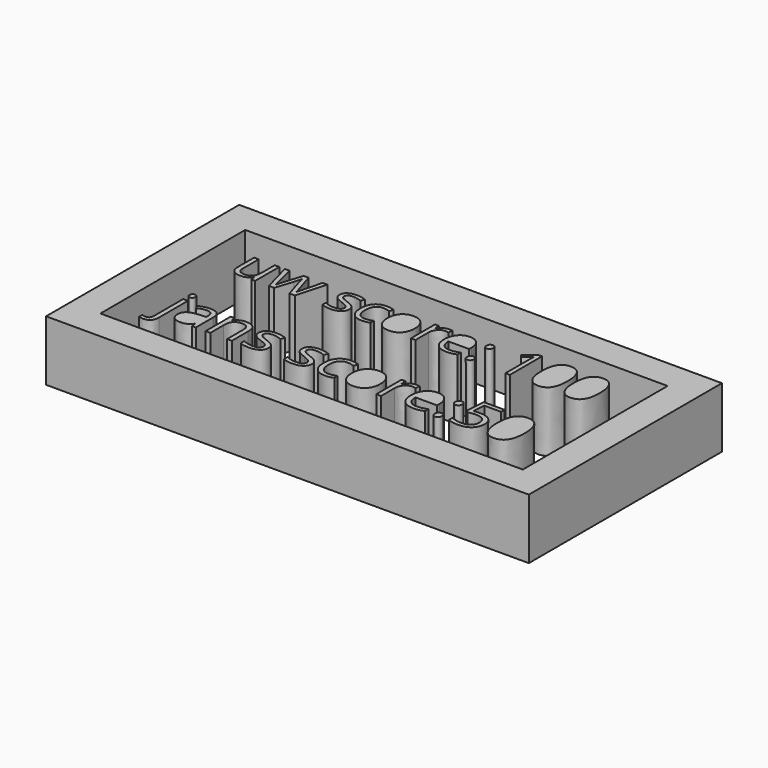
from build123d import *

# Parameters (mm, degrees)
F0_W           = 80
F0_H           = 40
F0_TEXT_SIZE   = 9.3251414556
F0_TEXT_SIZE_2 = 9.7321134399
F1_DEPTH       = 10


# Not quite as in the source:
# - Text() gives the source's letters only with a copy of the font that has no kerning and outlines rounded to 1/6400 em; it was checked with that copy


with BuildPart() as f1:
    # F0 (on Top) → F1 (new body)
    with BuildSketch(Plane.XY):
        with Locations((-35, -20.7777848959)):
            Rectangle(F0_W, F0_H)
        Polygon((-70, -20.7777848959), (-70, -5.7777848959), (0, -5.7777848959), (0, -20.7777848959), (0, -35.7777848959), (-70, -35.7777848959), align=None, mode=Mode.SUBTRACT)
        with BuildLine():
            add(Edge.make_bspline(
                [(-9.5991839217, -25.4409322699), (-9.9557746407, -26.1275024602), (-9.9557746407, -27.643583257)],
                knots=[0, 0, 0, 1, 1, 1], degree=2))
            add(Edge.make_bspline(
                [(-9.9557746407, -27.643583257), (-9.9557746407, -29.1596640539), (-9.5991839217, -29.8515564937)],
                knots=[0, 0, 0, 1, 1, 1], degree=2))
            add(Edge.make_bspline(
                [(-9.5991839217, -29.8515564937), (-9.2425932027, -30.5434489336), (-8.4640241275, -30.5434489336)],
                knots=[0, 0, 0, 1, 1, 1], degree=2))
            add(Edge.make_bspline(
                [(-8.4640241275, -30.5434489336), (-7.6748105533, -30.5434489336), (-7.3212611197, -29.8424326374)],
                knots=[0, 0, 0, 1, 1, 1], degree=2))
            add(Edge.make_bspline(
                [(-7.3212611197, -29.8424326374), (-6.9677116861, -29.1414163412), (-6.9677116861, -27.643583257)],
                knots=[0, 0, 0, 1, 1, 1], degree=2))
            add(Edge.make_bspline(
                [(-6.9677116861, -27.643583257), (-6.9677116861, -26.1472708156), (-7.3212611197, -25.4508164476)],
                knots=[0, 0, 0, 1, 1, 1], degree=2))
            add(Edge.make_bspline(
                [(-7.3212611197, -25.4508164476), (-7.6748105533, -24.7543620796), (-8.4640241275, -24.7543620796)],
                knots=[0, 0, 0, 1, 1, 1], degree=2))
            add(Edge.make_bspline(
                [(-8.4640241275, -24.7543620796), (-9.2425932027, -24.7543620796), (-9.5991839217, -25.4409322699)],
                knots=[0, 0, 0, 1, 1, 1], degree=2))
        make_face()
        with BuildLine():
            add(Edge.make_bspline(
                [(-14.2326185677, -10.6584024681), (-14.5742975789, -11.3162620568), (-14.5742975789, -12.7689442491)],
                knots=[0, 0, 0, 1, 1, 1], degree=2))
            add(Edge.make_bspline(
                [(-14.5742975789, -12.7689442491), (-14.5742975789, -14.2216264415), (-14.2326185677, -14.8845857169)],
                knots=[0, 0, 0, 1, 1, 1], degree=2))
            add(Edge.make_bspline(
                [(-14.2326185677, -14.8845857169), (-13.8909395566, -15.5475449922), (-13.1449282401, -15.5475449922)],
                knots=[0, 0, 0, 1, 1, 1], degree=2))
            add(Edge.make_bspline(
                [(-13.1449282401, -15.5475449922), (-12.3887175502, -15.5475449922), (-12.0499526458, -14.8758433968)],
                knots=[0, 0, 0, 1, 1, 1], degree=2))
            add(Edge.make_bspline(
                [(-12.0499526458, -14.8758433968), (-11.7111877413, -14.2041418013), (-11.7111877413, -12.7689442491)],
                knots=[0, 0, 0, 1, 1, 1], degree=2))
            add(Edge.make_bspline(
                [(-11.7111877413, -12.7689442491), (-11.7111877413, -11.3352037503), (-12.0499526458, -10.6678733149)],
                knots=[0, 0, 0, 1, 1, 1], degree=2))
            add(Edge.make_bspline(
                [(-12.0499526458, -10.6678733149), (-12.3887175502, -10.0005428795), (-13.1449282401, -10.0005428795)],
                knots=[0, 0, 0, 1, 1, 1], degree=2))
            add(Edge.make_bspline(
                [(-13.1449282401, -10.0005428795), (-13.8909395566, -10.0005428795), (-14.2326185677, -10.6584024681)],
                knots=[0, 0, 0, 1, 1, 1], degree=2))
        make_face()
        with BuildLine():
            add(Edge.make_bspline(
                [(-8.9012603511, -10.6584024681), (-9.2429393623, -11.3162620568), (-9.2429393623, -12.7689442491)],
                knots=[0, 0, 0, 1, 1, 1], degree=2))
            add(Edge.make_bspline(
                [(-9.2429393623, -12.7689442491), (-9.2429393623, -14.2216264415), (-8.9012603511, -14.8845857169)],
                knots=[0, 0, 0, 1, 1, 1], degree=2))
            add(Edge.make_bspline(
                [(-8.9012603511, -14.8845857169), (-8.55958134, -15.5475449922), (-7.8135700236, -15.5475449922)],
                knots=[0, 0, 0, 1, 1, 1], degree=2))
            add(Edge.make_bspline(
                [(-7.8135700236, -15.5475449922), (-7.0573593336, -15.5475449922), (-6.7185944292, -14.8758433968)],
                knots=[0, 0, 0, 1, 1, 1], degree=2))
            add(Edge.make_bspline(
                [(-6.7185944292, -14.8758433968), (-6.3798295248, -14.2041418013), (-6.3798295248, -12.7689442491)],
                knots=[0, 0, 0, 1, 1, 1], degree=2))
            add(Edge.make_bspline(
                [(-6.3798295248, -12.7689442491), (-6.3798295248, -11.3352037503), (-6.7185944292, -10.6678733149)],
                knots=[0, 0, 0, 1, 1, 1], degree=2))
            add(Edge.make_bspline(
                [(-6.7185944292, -10.6678733149), (-7.0573593336, -10.0005428795), (-7.8135700236, -10.0005428795)],
                knots=[0, 0, 0, 1, 1, 1], degree=2))
            add(Edge.make_bspline(
                [(-7.8135700236, -10.0005428795), (-8.55958134, -10.0005428795), (-8.9012603511, -10.6584024681)],
                knots=[0, 0, 0, 1, 1, 1], degree=2))
        make_face()
        with BuildLine():
            add(Edge.make_bspline(
                [(-32.9471323213, -27.0026323485), (-33.3417391084, -27.51128734), (-33.3417391084, -28.5179528239)],
                knots=[0, 0, 0, 1, 1, 1], degree=2))
            add(Edge.make_bspline(
                [(-33.3417391084, -28.5179528239), (-33.3417391084, -29.5170150942), (-32.9425703931, -30.0393558703)],
                knots=[0, 0, 0, 1, 1, 1], degree=2))
            add(Edge.make_bspline(
                [(-32.9425703931, -30.0393558703), (-32.5434016778, -30.5616966463), (-31.7693945308, -30.5616966463)],
                knots=[0, 0, 0, 1, 1, 1], degree=2))
            add(Edge.make_bspline(
                [(-31.7693945308, -30.5616966463), (-30.993866741, -30.5616966463), (-30.5924170616, -30.0416368344)],
                knots=[0, 0, 0, 1, 1, 1], degree=2))
            add(Edge.make_bspline(
                [(-30.5924170616, -30.0416368344), (-30.1909673822, -29.5215770224), (-30.1909673822, -28.5179528239)],
                knots=[0, 0, 0, 1, 1, 1], degree=2))
            add(Edge.make_bspline(
                [(-30.1909673822, -28.5179528239), (-30.1909673822, -27.5249731245), (-30.5924170616, -27.0094752407)],
                knots=[0, 0, 0, 1, 1, 1], degree=2))
            add(Edge.make_bspline(
                [(-30.5924170616, -27.0094752407), (-30.993866741, -26.4939773569), (-31.7785183871, -26.4939773569)],
                knots=[0, 0, 0, 1, 1, 1], degree=2))
            add(Edge.make_bspline(
                [(-31.7785183871, -26.4939773569), (-32.5525255341, -26.4939773569), (-32.9471323213, -27.0026323485)],
                knots=[0, 0, 0, 1, 1, 1], degree=2))
        make_face()
        with BuildLine():
            add(Edge.make_bspline(
                [(-39.0272954661, -12.1547962611), (-39.4054008111, -12.6421806075), (-39.4054008111, -13.6067499268)],
                knots=[0, 0, 0, 1, 1, 1], degree=2))
            add(Edge.make_bspline(
                [(-39.4054008111, -13.6067499268), (-39.4054008111, -14.5640339793), (-39.0229243061, -15.0645318059)],
                knots=[0, 0, 0, 1, 1, 1], degree=2))
            add(Edge.make_bspline(
                [(-39.0229243061, -15.0645318059), (-38.6404478011, -15.5650296325), (-37.8988076447, -15.5650296325)],
                knots=[0, 0, 0, 1, 1, 1], degree=2))
            add(Edge.make_bspline(
                [(-37.8988076447, -15.5650296325), (-37.1557104349, -15.5650296325), (-36.7710483499, -15.0667173859)],
                knots=[0, 0, 0, 1, 1, 1], degree=2))
            add(Edge.make_bspline(
                [(-36.7710483499, -15.0667173859), (-36.3863862648, -14.5684051394), (-36.3863862648, -13.6067499268)],
                knots=[0, 0, 0, 1, 1, 1], degree=2))
            add(Edge.make_bspline(
                [(-36.3863862648, -13.6067499268), (-36.3863862648, -12.6552940876), (-36.7710483499, -12.1613530012)],
                knots=[0, 0, 0, 1, 1, 1], degree=2))
            add(Edge.make_bspline(
                [(-36.7710483499, -12.1613530012), (-37.1557104349, -11.6674119147), (-37.9075499648, -11.6674119147)],
                knots=[0, 0, 0, 1, 1, 1], degree=2))
            add(Edge.make_bspline(
                [(-37.9075499648, -11.6674119147), (-38.6491901212, -11.6674119147), (-39.0272954661, -12.1547962611)],
                knots=[0, 0, 0, 1, 1, 1], degree=2))
        make_face()
        with BuildLine():
            add(Edge.make_bspline(
                [(-61.0052715614, -30.3480463434), (-60.7467622982, -30.5708205027), (-60.2814456244, -30.5708205027)],
                knots=[0, 0, 0, 1, 1, 1], degree=2))
            add(Edge.make_bspline(
                [(-60.2814456244, -30.5708205027), (-59.5439339027, -30.5708205027), (-59.1234761893, -30.1670898592)],
                knots=[0, 0, 0, 1, 1, 1], degree=2))
            add(Edge.make_bspline(
                [(-59.1234761893, -30.1670898592), (-58.7030184758, -29.7633592157), (-58.7030184758, -29.0364919931)],
                knots=[0, 0, 0, 1, 1, 1], degree=2))
            Line((-58.7030184758, -29.0364919931), (-58.7030184758, -28.5666133911))
            Line((-58.7030184758, -28.5666133911), (-59.4922320501, -28.5985468883))
            add(Edge.make_bspline(
                [(-59.4922320501, -28.5985468883), (-60.4335098968, -28.6320010283), (-60.8486453608, -28.8912706129)],
                knots=[0, 0, 0, 1, 1, 1], degree=2))
            add(Edge.make_bspline(
                [(-60.8486453608, -28.8912706129), (-61.2637808247, -29.1505401975), (-61.2637808247, -29.6964509358)],
                knots=[0, 0, 0, 1, 1, 1], degree=2))
            add(Edge.make_bspline(
                [(-61.2637808247, -29.6964509358), (-61.2637808247, -30.1252721842), (-61.0052715614, -30.3480463434)],
                knots=[0, 0, 0, 1, 1, 1], degree=2))
        make_face()
        with BuildLine():
            add(Edge.make_bspline(
                [(-21.0800364954, -26.8817412518), (-21.4122969308, -26.4848535006), (-22.0311985199, -26.4848535006)],
                knots=[0, 0, 0, 1, 1, 1], degree=2))
            add(Edge.make_bspline(
                [(-22.0311985199, -26.4848535006), (-22.6577033226, -26.4848535006), (-23.0310211116, -26.8931460723)],
                knots=[0, 0, 0, 1, 1, 1], degree=2))
            add(Edge.make_bspline(
                [(-23.0310211116, -26.8931460723), (-23.4043389006, -27.3014386439), (-23.4712471805, -28.0237439383)],
                knots=[0, 0, 0, 1, 1, 1], degree=2))
            Line((-23.4712471805, -28.0237439383), (-20.74777606, -28.0237439383))
            add(Edge.make_bspline(
                [(-20.74777606, -28.0237439383), (-20.74777606, -27.278629003), (-21.0800364954, -26.8817412518)],
                knots=[0, 0, 0, 1, 1, 1], degree=2))
        make_face()
        with BuildLine():
            add(Edge.make_bspline(
                [(-27.6564511037, -12.0389605196), (-27.9748172612, -11.6586695946), (-28.5678379757, -11.6586695946)],
                knots=[0, 0, 0, 1, 1, 1], degree=2))
            add(Edge.make_bspline(
                [(-28.5678379757, -11.6586695946), (-29.1681439569, -11.6586695946), (-29.5258505549, -12.0498884197)],
                knots=[0, 0, 0, 1, 1, 1], degree=2))
            add(Edge.make_bspline(
                [(-29.5258505549, -12.0498884197), (-29.8835571529, -12.4411072448), (-29.9476675004, -13.1332075872)],
                knots=[0, 0, 0, 1, 1, 1], degree=2))
            Line((-29.9476675004, -13.1332075872), (-27.3380849462, -13.1332075872))
            add(Edge.make_bspline(
                [(-27.3380849462, -13.1332075872), (-27.3380849462, -12.4192514445), (-27.6564511037, -12.0389605196)],
                knots=[0, 0, 0, 1, 1, 1], degree=2))
        make_face()
        with Locations((-65, -16.1070534796)):
            Text('uw score: 100', F0_TEXT_SIZE, font='Open Sans', text_align=(TextAlign.LEFT, TextAlign.BOTTOM))
        with Locations((-65, -31.12737574)):
            Text('jans score:50', F0_TEXT_SIZE_2, font='Open Sans', text_align=(TextAlign.LEFT, TextAlign.BOTTOM))
    extrude(amount=F1_DEPTH)


solid = f1.part
